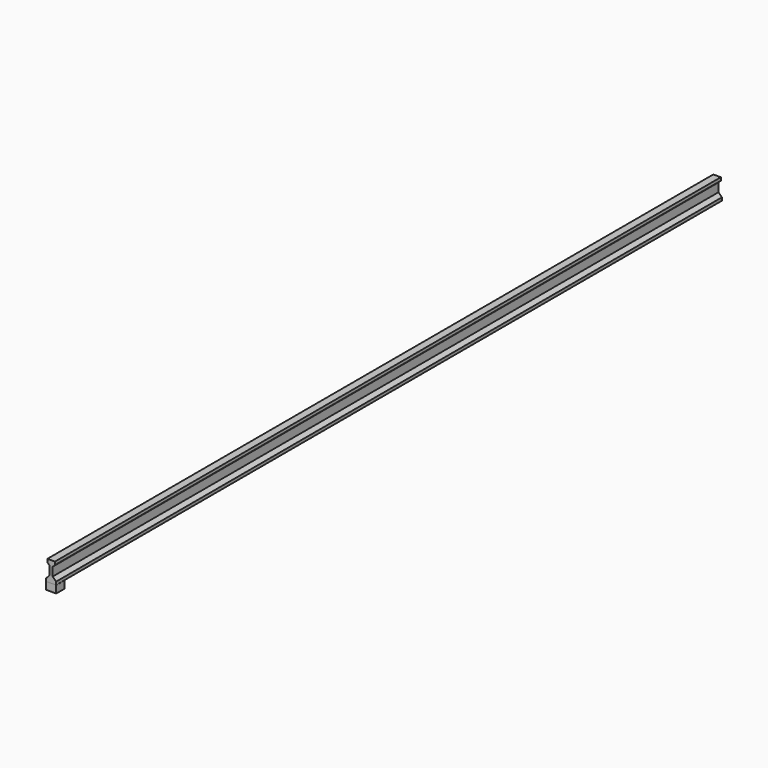
from build123d import *

# Parameters (mm, degrees)
F1_DEPTH = 56200
F3_W     = 660.4
F3_H     = 683
F4_DEPTH = 500
F3_W_2   = 11.3
F5_DEPTH = 500
F6_DEPTH = 500


with BuildPart() as f1:
    # F0 (on Front) → F1 (new body)
    with BuildSketch(Plane.XZ):
        Polygon((254, 759.618646022), (0, 759.618646022), (-254, 759.618646022), (-258.8367380354, 556.47621824), (-101.6, 404.07621824), (-101.6, -180.12378176), (-330.2, -408.72378176), (-330.2, -611.92378176), (0, -611.92378176), (330.2, -611.92378176), (330.2, -408.72378176), (101.6, -180.12378176), (101.6, 404.07621824), (258.8367380354, 556.47621824), align=None)
    extrude(amount=F1_DEPTH)


with BuildPart() as f4:
    # F3 (on face) → F4 (new body)
    with BuildSketch(Plane(origin=(0, 0, -611.92378176), x_dir=(1, 0, 0), z_dir=(0, 0, -1))):
        with Locations((0, 55858.5)):
            Rectangle(F3_W, F3_H)
    extrude(amount=F4_DEPTH)

    # F3 (on face) → F5 (join)
    with BuildSketch(Plane(origin=(0, 0, -611.92378176), x_dir=(1, 0, 0), z_dir=(0, 0, -1))):
        with Locations((335.85, 55858.5)):
            Rectangle(F3_W_2, F3_H)
    extrude(amount=F5_DEPTH)

    # F3 (on face) → F6 (join)
    with BuildSketch(Plane(origin=(0, 0, -611.92378176), x_dir=(1, 0, 0), z_dir=(0, 0, -1))):
        with Locations((-335.85, 55858.5)):
            Rectangle(F3_W_2, F3_H)
    extrude(amount=F6_DEPTH)


solid = Compound([f1.part, f4.part])
